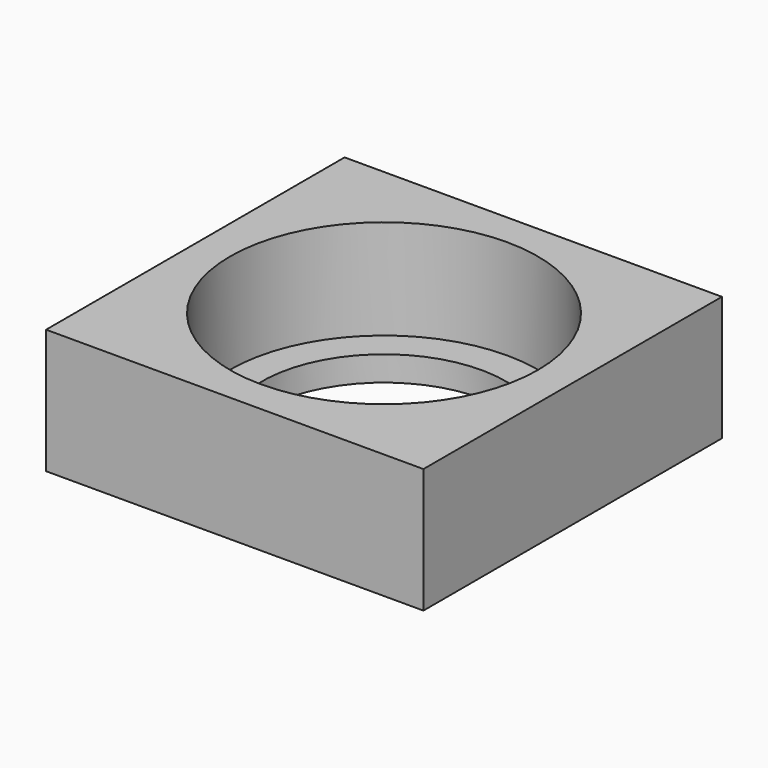
from build123d import *

# Parameters (mm, degrees)
F0_W     = 38.4559035301
F0_H     = 38.0239486694
F1_DEPTH = 12.7
F2_R     = 15.6804316887
F5_DEPTH = 10.16
F6_R     = 12.442666724
F7_DEPTH = 12.701


# Not quite as in the source:
# - the program builds the solid bodies; features that only make, move or delete a surface that nothing else refers to are left out


with BuildPart() as f1:
    # F0 (on Top) → F1 (new body)
    with BuildSketch(Plane.XY):
        with Locations((19.2279517651, 19.0119743347)):
            Rectangle(F0_W, F0_H)
    extrude(amount=F1_DEPTH)

    # F2 (on face) → F5 (cut)
    with BuildSketch(Plane.XY.offset(12.7)):
        with Locations((19.2279517651, 19.0119743347)):
            Circle(F2_R)
    extrude(amount=-F5_DEPTH, mode=Mode.SUBTRACT)

    # F6 (on face) → F7 (cut, through all)
    with BuildSketch(Plane(origin=(0, 0, 0), x_dir=(1, 0, 0), z_dir=(0, 0, -1))):
        with Locations((19.2279517651, -19.0119743347)):
            Circle(F6_R)
    extrude(amount=-F7_DEPTH, mode=Mode.SUBTRACT)


solid = f1.part
